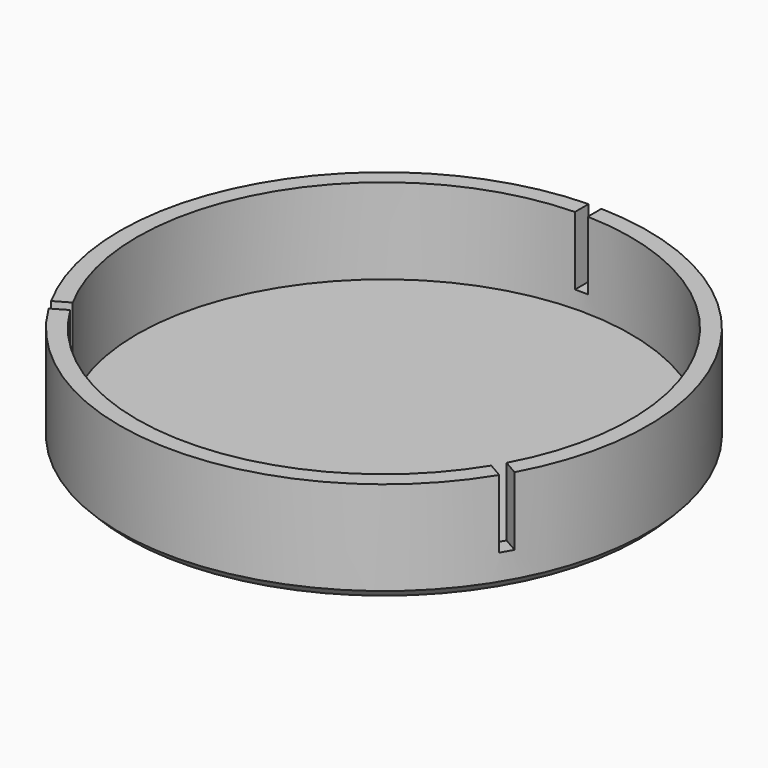
from build123d import *

# Parameters (mm, degrees)
F3_W            = 1.5
F3_H            = 4.2986176481
F4_DEPTH        = 8
F4_COPIES_COUNT = 3
F5_SIZE         = 1


# Not quite as in the source:
# - a pattern or mirror of a feature is missing from the dataset's text; its kind, count and spacing are read off the source's solid


with BuildPart() as f1:
    # F0 (on Front) → F1 (revolve)
    with BuildSketch(Plane.XZ):
        Polygon((-30.9, 0), (0, 0), (0, 2), (-28.9, 2), (-28.9, 12), (-30.9, 12), align=None)
    revolve(axis=Axis((0, 0, 1), (0, 0, -1)))

    # F3 (on offset) → F4 (cut)
    with BuildSketch(Plane.XY.offset(12)):
        with Locations((0, 29.3811720078)):
            Rectangle(F3_W, F3_H)
    f4 = extrude(amount=-F4_DEPTH, mode=Mode.SUBTRACT)

    # F4_copies: F4 ×3 about axis
    f4_copies_axis = Axis((0, 0, 0), (0, 0, 1))
    for i in range(1, F4_COPIES_COUNT):
        add(f4.rotate(f4_copies_axis, i * 360 / F4_COPIES_COUNT), mode=Mode.SUBTRACT)

    # F5
    f5_edges = [f1.edges().sort_by_distance(p)[0] for p in [
        (30.9, 0, 0),
    ]]
    chamfer(f5_edges, length=F5_SIZE)


solid = f1.part
